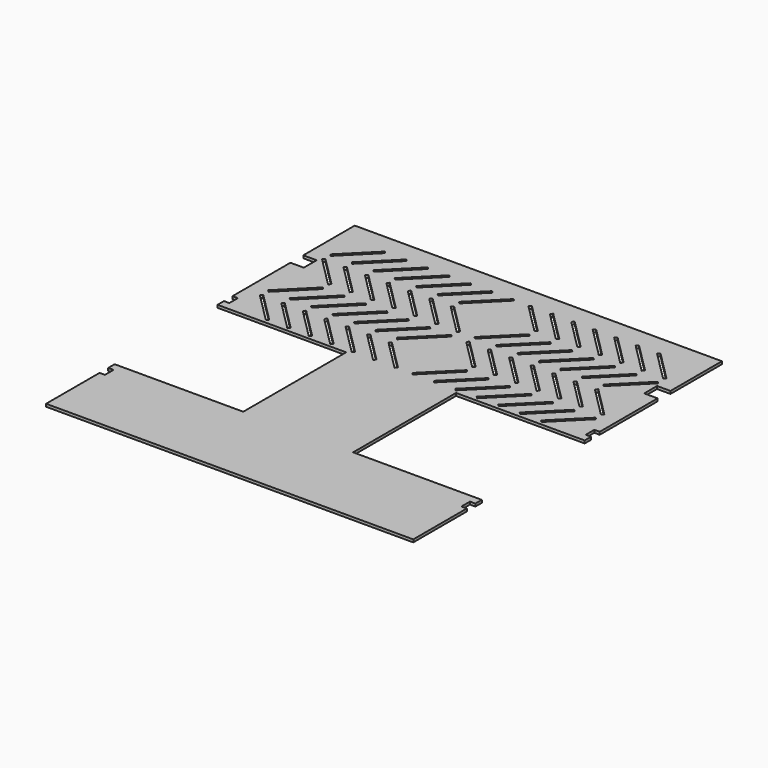
from build123d import *

# Parameters (mm, degrees)
F1_DEPTH = 3.175


# Not quite as in the source:
# - a length typed as a fraction of an inch, garbled in the dataset ("3 / 203.2 mm" for 3/8 in), is restored


with BuildPart() as f1:
    # F0 (on Top) → F1 (new body)
    with BuildSketch(Plane.XY):
        Polygon((-217.4873984, -149.3041718), (-217.4873984, -228.5206758), (217.4874238, -228.5206758), (217.4874238, -149.3041718), (211.1374238, -149.3041718), (211.1374238, -136.6041718), (217.4874238, -136.6041718), (217.4874238, -127.0791718), (65.0874238, -127.0791718), (65.0874238, 25.3208282), (217.4874238, 25.3208282), (217.4874238, 34.8458282), (211.1374238, 34.8458282), (211.1374238, 47.5458282), (217.4874238, 47.5458282), (217.4874238, 133.2706758), (201.6124238, 133.2706758), (201.6124238, 152.3208282), (217.4874238, 152.3206758), (217.4874238, 228.5206758), (-217.4873984, 228.5206758), (-217.4873984, 152.3206758), (-201.6123984, 152.3206758), (-201.6123984, 133.2706758), (-217.4873984, 133.2706758), (-217.4873984, 47.5458282), (-211.1373984, 47.5458282), (-211.1373984, 34.8458282), (-217.4873984, 34.8458282), (-217.4873984, 25.3208282), (-65.0873984, 25.3208282), (-65.0873984, -127.0791718), (-217.4873984, -127.0791718), (-217.4873984, -136.6041718), (-211.1373984, -136.6041718), (-211.1373984, -149.3041718), align=None)
        Polygon((-199.1054184, 65.0193518), (-196.8602362, 67.264534), (-160.9392514, 31.3433714), (-163.1844336, 29.0983924), align=None, mode=Mode.SUBTRACT)
        Polygon((-173.7054184, 65.0193518), (-171.4602362, 67.264534), (-135.5392514, 31.3433714), (-137.7844336, 29.0983924), align=None, mode=Mode.SUBTRACT)
        Polygon((-148.3054184, 65.0193518), (-146.0602362, 67.264534), (-110.1392514, 31.3433714), (-112.3844336, 29.0983924), align=None, mode=Mode.SUBTRACT)
        Polygon((-160.9392514, 111.0566994), (-196.8602362, 75.1355368), (-199.1054184, 77.380719), (-163.1844336, 113.3016784), align=None, mode=Mode.SUBTRACT)
        Polygon((-135.5392514, 111.0566994), (-171.4602362, 75.1355368), (-173.7054184, 77.380719), (-137.7844336, 113.3016784), align=None, mode=Mode.SUBTRACT)
        Polygon((-110.1392514, 111.0566994), (-146.0602362, 75.1355368), (-148.3054184, 77.380719), (-112.3844336, 113.3016784), align=None, mode=Mode.SUBTRACT)
        Polygon((-122.9054184, 65.0193518), (-120.6602362, 67.264534), (-84.7392514, 31.3433714), (-86.9844336, 29.0983924), align=None, mode=Mode.SUBTRACT)
        Polygon((-97.5054184, 65.0193518), (-95.2602362, 67.264534), (-59.3392514, 31.3433714), (-61.5844336, 29.0983924), align=None, mode=Mode.SUBTRACT)
        Polygon((-72.1054184, 65.0193518), (-69.8602362, 67.264534), (-33.9392514, 31.3433714), (-36.1844336, 29.0983924), align=None, mode=Mode.SUBTRACT)
        Polygon((-46.7054184, 65.0193518), (-44.4602362, 67.264534), (-8.5392514, 31.3433714), (-10.7844336, 29.0983924), align=None, mode=Mode.SUBTRACT)
        Polygon((-84.7392514, 111.0566994), (-120.6602362, 75.1355368), (-122.9054184, 77.380719), (-86.9844336, 113.3016784), align=None, mode=Mode.SUBTRACT)
        Polygon((-59.3392514, 111.0566994), (-95.2602362, 75.1355368), (-97.5054184, 77.380719), (-61.5844336, 113.3016784), align=None, mode=Mode.SUBTRACT)
        Polygon((-33.9392514, 111.0566994), (-69.8602362, 75.1355368), (-72.1054184, 77.380719), (-36.1844336, 113.3016784), align=None, mode=Mode.SUBTRACT)
        Polygon((-8.5392514, 111.0566994), (-44.4602362, 75.1355368), (-46.7054184, 77.380719), (-10.7844336, 113.3016784), align=None, mode=Mode.SUBTRACT)
        Polygon((-199.1054184, 157.0943518), (-196.8602362, 159.339534), (-160.9392514, 123.4183714), (-163.1844336, 121.1733924), align=None, mode=Mode.SUBTRACT)
        Polygon((-173.7054184, 157.0943518), (-171.4602362, 159.339534), (-135.5392514, 123.4183714), (-137.7844336, 121.1733924), align=None, mode=Mode.SUBTRACT)
        Polygon((-148.3054184, 157.0943518), (-146.0602362, 159.339534), (-110.1392514, 123.4183714), (-112.3844336, 121.1733924), align=None, mode=Mode.SUBTRACT)
        Polygon((-160.9392514, 203.1316994), (-196.8602362, 167.2105368), (-199.1054184, 169.455719), (-163.1844336, 205.3766784), align=None, mode=Mode.SUBTRACT)
        Polygon((-135.5392514, 203.1316994), (-171.4602362, 167.2105368), (-173.7054184, 169.455719), (-137.7844336, 205.3766784), align=None, mode=Mode.SUBTRACT)
        Polygon((-110.1392514, 203.1316994), (-146.0602362, 167.2105368), (-148.3054184, 169.455719), (-112.3844336, 205.3766784), align=None, mode=Mode.SUBTRACT)
        Polygon((-122.9054184, 157.0943518), (-120.6602362, 159.339534), (-84.7392514, 123.4183714), (-86.9844336, 121.1733924), align=None, mode=Mode.SUBTRACT)
        Polygon((-97.5054184, 157.0943518), (-95.2602362, 159.339534), (-59.3392514, 123.4183714), (-61.5844336, 121.1733924), align=None, mode=Mode.SUBTRACT)
        Polygon((-72.1054184, 157.0943518), (-69.8602362, 159.339534), (-33.9392514, 123.4183714), (-36.1844336, 121.1733924), align=None, mode=Mode.SUBTRACT)
        Polygon((-46.7054184, 157.0943518), (-44.4602362, 159.339534), (-8.5392514, 123.4183714), (-10.7844336, 121.1733924), align=None, mode=Mode.SUBTRACT)
        Polygon((-84.7392514, 203.1316994), (-120.6602362, 167.2105368), (-122.9054184, 169.455719), (-86.9844336, 205.3766784), align=None, mode=Mode.SUBTRACT)
        Polygon((-59.3392514, 203.1316994), (-95.2602362, 167.2105368), (-97.5054184, 169.455719), (-61.5844336, 205.3766784), align=None, mode=Mode.SUBTRACT)
        Polygon((-33.9392514, 203.1316994), (-69.8602362, 167.2105368), (-72.1054184, 169.455719), (-36.1844336, 205.3766784), align=None, mode=Mode.SUBTRACT)
        Polygon((-8.5392514, 203.1316994), (-44.4602362, 167.2105368), (-46.7054184, 169.455719), (-10.7844336, 205.3766784), align=None, mode=Mode.SUBTRACT)
        Polygon((44.4602616, 67.2641784), (46.705774, 65.0190216), (10.784459, 29.0980368), (8.5396324, 31.343219), align=None, mode=Mode.SUBTRACT)
        Polygon((69.8602616, 67.2641784), (72.105774, 65.0190216), (36.184459, 29.0980368), (33.9396324, 31.343219), align=None, mode=Mode.SUBTRACT)
        Polygon((95.2602616, 67.2641784), (97.505774, 65.0190216), (61.584459, 29.0980368), (59.3396324, 31.343219), align=None, mode=Mode.SUBTRACT)
        Polygon((120.6602616, 67.2641784), (122.905774, 65.0190216), (86.984459, 29.0980368), (84.7396324, 31.343219), align=None, mode=Mode.SUBTRACT)
        Polygon((10.784459, 113.302034), (46.705774, 77.3810492), (44.4602616, 75.1358924), (8.5396324, 111.0568518), align=None, mode=Mode.SUBTRACT)
        Polygon((36.184459, 113.302034), (72.105774, 77.3810492), (69.8602616, 75.1358924), (33.9396324, 111.0568518), align=None, mode=Mode.SUBTRACT)
        Polygon((61.584459, 113.302034), (97.505774, 77.3810492), (95.2602616, 75.1358924), (59.3396324, 111.0568518), align=None, mode=Mode.SUBTRACT)
        Polygon((86.984459, 113.302034), (122.905774, 77.3810492), (120.6602616, 75.1358924), (84.7396324, 111.0568518), align=None, mode=Mode.SUBTRACT)
        Polygon((146.0602616, 67.2641784), (148.305774, 65.0190216), (112.384459, 29.0980368), (110.1396324, 31.343219), align=None, mode=Mode.SUBTRACT)
        Polygon((171.4602616, 67.2641784), (173.705774, 65.0190216), (137.784459, 29.0980368), (135.5396324, 31.343219), align=None, mode=Mode.SUBTRACT)
        Polygon((196.8602616, 67.2641784), (199.105774, 65.0190216), (163.184459, 29.0980368), (160.9396324, 31.343219), align=None, mode=Mode.SUBTRACT)
        Polygon((112.384459, 113.302034), (148.305774, 77.3810492), (146.0602616, 75.1358924), (110.1396324, 111.0568518), align=None, mode=Mode.SUBTRACT)
        Polygon((137.784459, 113.302034), (173.705774, 77.3810492), (171.4602616, 75.1358924), (135.5396324, 111.0568518), align=None, mode=Mode.SUBTRACT)
        Polygon((163.184459, 113.302034), (199.105774, 77.3810492), (196.8602616, 75.1358924), (160.9396324, 111.0568518), align=None, mode=Mode.SUBTRACT)
        Polygon((44.4602616, 159.3391784), (46.705774, 157.0940216), (10.784459, 121.1730368), (8.5396324, 123.418219), align=None, mode=Mode.SUBTRACT)
        Polygon((69.8602616, 159.3391784), (72.105774, 157.0940216), (36.184459, 121.1730368), (33.9396324, 123.418219), align=None, mode=Mode.SUBTRACT)
        Polygon((95.2602616, 159.3391784), (97.505774, 157.0940216), (61.584459, 121.1730368), (59.3396324, 123.418219), align=None, mode=Mode.SUBTRACT)
        Polygon((120.6602616, 159.3391784), (122.905774, 157.0940216), (86.984459, 121.1730368), (84.7396324, 123.418219), align=None, mode=Mode.SUBTRACT)
        Polygon((10.784459, 205.377034), (46.705774, 169.4560492), (44.4602616, 167.2108924), (8.5396324, 203.1318518), align=None, mode=Mode.SUBTRACT)
        Polygon((36.184459, 205.377034), (72.105774, 169.4560492), (69.8602616, 167.2108924), (33.9396324, 203.1318518), align=None, mode=Mode.SUBTRACT)
        Polygon((61.584459, 205.377034), (97.505774, 169.4560492), (95.2602616, 167.2108924), (59.3396324, 203.1318518), align=None, mode=Mode.SUBTRACT)
        Polygon((86.984459, 205.377034), (122.905774, 169.4560492), (120.6602616, 167.2108924), (84.7396324, 203.1318518), align=None, mode=Mode.SUBTRACT)
        Polygon((146.0602616, 159.3391784), (148.305774, 157.0940216), (112.384459, 121.1730368), (110.1396324, 123.418219), align=None, mode=Mode.SUBTRACT)
        Polygon((171.4602616, 159.3391784), (173.705774, 157.0940216), (137.784459, 121.1730368), (135.5396324, 123.418219), align=None, mode=Mode.SUBTRACT)
        Polygon((196.8602616, 159.3391784), (199.105774, 157.0940216), (163.184459, 121.1730368), (160.9396324, 123.418219), align=None, mode=Mode.SUBTRACT)
        Polygon((112.384459, 205.377034), (148.305774, 169.4560492), (146.0602616, 167.2108924), (110.1396324, 203.1318518), align=None, mode=Mode.SUBTRACT)
        Polygon((137.784459, 205.377034), (173.705774, 169.4560492), (171.4602616, 167.2108924), (135.5396324, 203.1318518), align=None, mode=Mode.SUBTRACT)
        Polygon((163.184459, 205.377034), (199.105774, 169.4560492), (196.8602616, 167.2108924), (160.9396324, 203.1318518), align=None, mode=Mode.SUBTRACT)
    extrude(amount=F1_DEPTH)


solid = f1.part
